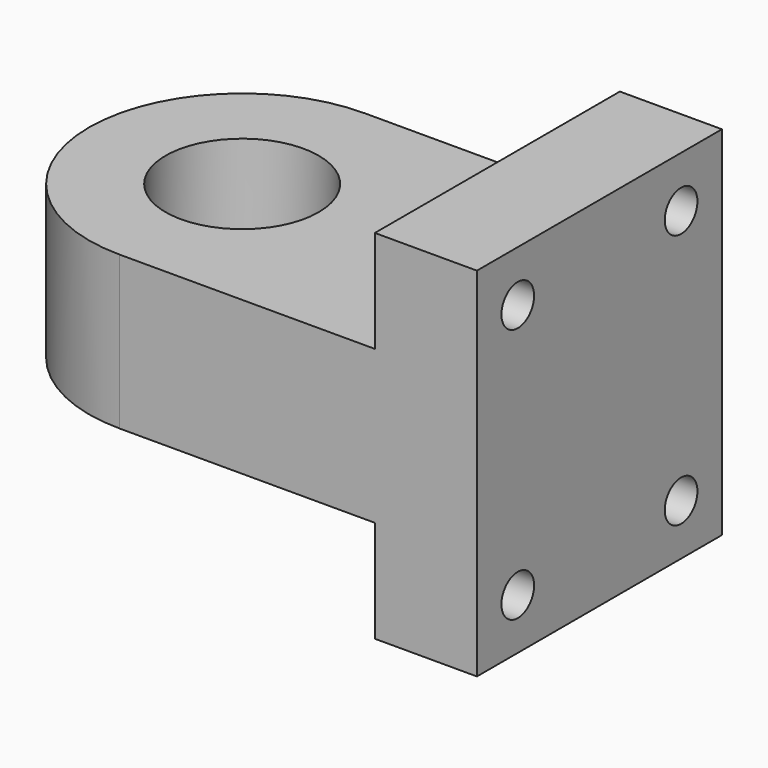
from build123d import *

# Parameters (mm, degrees)
F1_DEPTH = 30
F2_R     = 30
F3_R     = 29.99999
F4_R     = 15
F5_DEPTH = 25
F7_R     = 4
F8_DEPTH = 20


# Not quite as in the source:
# - a fillet or chamfer is up to 0.001 mm smaller than in the source, because OpenCascade refuses the exact size


with BuildPart() as f1:
    # F0 (on Front) → F1 (new body, symmetric)
    with BuildSketch(Plane.XZ):
        Polygon((-100, 0), (0, 0), (0, 35), (-20, 35), (-20, 15), (-100, 15), align=None)
    extrude(amount=F1_DEPTH, both=True)

    # F2
    f2_edges = [f1.edges().sort_by_distance(p)[0] for p in [
        (-100, -30, 7.5),
    ]]
    fillet(f2_edges, radius=F2_R)

    # F3 (radius 30 in the source; OpenCascade refuses exactly that, so slightly less here)
    f3_edges = [f1.edges().sort_by_distance(p)[0] for p in [
        (-100, 30, 7.5),
    ]]
    fillet(f3_edges, radius=F3_R)

    # F4 (on face) → F5 (cut)
    with BuildSketch(Plane.XY.offset(15)):
        with Locations((-70, 0)):
            Circle(F4_R)
    extrude(amount=-F5_DEPTH, mode=Mode.SUBTRACT)

    # F6: F1 across plane


with BuildPart() as f1_1:
    add(f1.part)
    add(f1.part.mirror(Plane.XY))

    # F7 (on face) → F8 (cut, through all)
    with BuildSketch(Plane.YZ):
        with BuildLine():
            ThreePointArc((-24, -25), (-20, -29), (-16, -25))
            ThreePointArc((-16, -25), (-20, -21), (-24, -25))
        make_face()
        with Locations((-20, 25)):
            Circle(F7_R)
        with Locations((20, -25)):
            Circle(F7_R)
        with Locations((20, 25)):
            Circle(F7_R)
    extrude(amount=-F8_DEPTH, mode=Mode.SUBTRACT)


solid = f1_1.part
